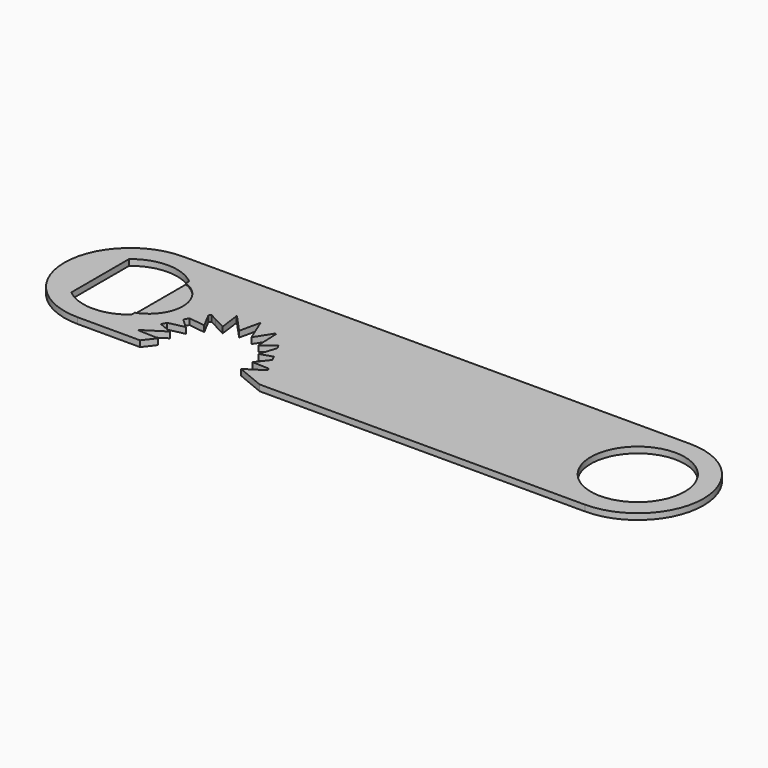
from build123d import *

# Parameters (mm, degrees)
F0_R     = 15.875
F1_DEPTH = 1.016
F3_DEPTH = 0.381


# Not quite as in the source:
# - a pattern or mirror of a feature is missing from the dataset's text; its kind, count and spacing are read off the source's solid
# - a feature names something its author has since deleted; it is built from what else it names


with BuildPart() as f1:
    # F0 (on Top) → F1 (new body, symmetric)
    with BuildSketch(Plane.XY):
        with BuildLine():
            Line((76.2, 22.225), (-95.25, 22.225))
            ThreePointArc((-95.25, 22.225), (-117.475, 0), (-95.25, -22.225))
            Line((-95.25, -22.225), (-81.2163393225, -22.225))
            Line((-81.2163393225, -22.225), (-80.4999828905, -20.8488920975))
            Line((-80.4999828905, -20.8488920975), (-81.8859980281, -17.8765730428))
            Line((-81.8859980281, -17.8765730428), (-80.3221061469, -17.944854037))
            Line((-80.3221061469, -17.944854037), (-81.0788131138, -9.2956538274))
            Line((-81.0788131138, -9.2956538274), (-79.6325889287, -9.8946994991))
            Line((-79.6325889287, -9.8946994991), (-77.3854601863, -1.5083008612))
            Line((-77.3854601863, -1.5083008612), (-76.231339678, -2.5658574615))
            Line((-76.231339678, -2.5658574615), (-71.2514121167, 4.5462161589))
            Line((-71.2514121167, 4.5462161589), (-70.5285992516, 3.1577055639))
            Line((-70.5285992516, 3.1577055639), (-63.4165256312, 8.1376331253))
            Line((-63.4165256312, 8.1376331253), (-63.2122023083, 6.5856434055))
            Line((-63.2122023083, 6.5856434055), (-54.8258036704, 8.832772148))
            Line((-54.8258036704, 8.832772148), (-55.1646142981, 7.3044961686))
            Line((-55.1646142981, 7.3044961686), (-46.5154140885, 6.5477892017))
            Line((-46.5154140885, 6.5477892017), (-47.3564931047, 5.2275596009))
            Line((-47.3564931047, 5.2275596009), (-39.4877125173, 1.5582869527))
            Line((-39.4877125173, 1.5582869527), (-40.7296133796, 0.6053429047))
            Line((-40.7296133796, 0.6053429047), (-34.5903434842, -5.5339269908))
            Line((-34.5903434842, -5.5339269908), (-36.0832746201, -6.0046463698))
            Line((-36.0832746201, -6.0046463698), (-32.4140019719, -13.8734269572))
            Line((-32.4140019719, -13.8734269572), (-33.9778938531, -13.805145963))
            Line((-33.9778938531, -13.805145963), (-33.273088024, -21.8611134529))
            Line((-33.273088024, -21.8611134529), (-33.0836606775, -22.225))
            Line((-33.0836606775, -22.225), (76.2, -22.225))
            ThreePointArc((76.2, -22.225), (98.425, 0), (76.2, 22.225))
        make_face()
        with BuildLine():
            ThreePointArc((-105.41, 12.1979516723), (-95.25, 15.875), (-85.09, 12.1979516723))
            Line((-85.09, 12.1979516723), (-85.09, -12.1979516723))
            ThreePointArc((-85.09, -12.1979516723), (-95.25, -15.875), (-105.41, -12.1979516723))
            Line((-105.41, -12.1979516723), (-105.41, 12.1979516723))
        make_face(mode=Mode.SUBTRACT)
        with Locations((76.2, 0)):
            Circle(F0_R, mode=Mode.SUBTRACT)
        Polygon((-80.4999828905, -20.8488920975), (-81.2163393225, -22.225), (-79.8582932371, -22.225), align=None)
        Polygon((-33.2412520763, -22.225), (-33.0836606775, -22.225), (-33.273088024, -21.8611134529), align=None)
        Polygon((-80.4999828905, -20.8488920975), (-79.8582932371, -22.225), (-77.6369016412, -22.225), (-74.1351559236, -22.225), (-71.1579054788, -18.3449716791), (-78.4147248097, -18.0281321046), (-79.3376725148, -18.6161146398), align=None)
        Polygon((-81.8859980281, -17.8765730428), (-80.4999828905, -20.8488920975), (-79.3376725148, -18.6161146398), (-80.2145068425, -19.1747197137), (-80.3221061469, -17.944854037), align=None)
        Polygon((-33.7748775265, -22.225), (-33.2412520763, -22.225), (-33.273088024, -21.8611134529), (-37.1054537581, -14.4992073738), (-43.1420945212, -18.3449716791), align=None)
        Polygon((-37.1054537581, -14.4992073738), (-33.273088024, -21.8611134529), (-33.9778938531, -13.805145963), (-35.8852751903, -13.7218678954), align=None)
        Polygon((-79.0178794125, -18.001797806), (-79.3376725148, -18.6161146398), (-78.4147248097, -18.0281321046), align=None)
        Polygon((-80.2145068425, -19.1747197137), (-79.3376725148, -18.6161146398), (-79.0178794125, -18.001797806), (-80.3221061469, -17.944854037), align=None)
        Polygon((-35.8852751903, -13.7218678954), (-33.9778938531, -13.805145963), (-34.0854931575, -12.5752802863), align=None)
        Polygon((-34.0854931575, -12.5752802863), (-33.9778938531, -13.805145963), (-32.4140019719, -13.8734269572), (-36.0832746201, -6.0046463698), (-37.9041095643, -6.5787534225), (-39.8848289883, -9.1600772324), (-37.5478999587, -13.6492761303), (-35.8852751903, -13.7218678954), align=None)
        Polygon((-37.5478999587, -13.6492761303), (-37.1054537581, -14.4992073738), (-35.8852751903, -13.7218678954), align=None)
        Polygon((-81.0788131138, -9.2956538274), (-80.3221061469, -17.944854037), (-79.0178794125, -18.001797806), (-75.6552159218, -11.5421813412), (-77.8687195378, -10.6253181231), (-79.9521174914, -11.0871963296), (-79.6325889287, -9.8946994991), align=None)
        Polygon((-79.0178794125, -18.001797806), (-78.4147248097, -18.0281321046), (-71.1579054788, -13.4050283209), (-75.6552159218, -11.5421813412), align=None)
        Polygon((-43.1420945212, -13.4050283209), (-37.5478999587, -13.6492761303), (-39.8848289883, -9.1600772324), align=None)
        Polygon((-77.8687195378, -10.6253181231), (-75.6552159218, -11.5421813412), (-74.8268774652, -9.950957971), align=None)
        Polygon((-37.9041095643, -6.5787534225), (-36.0832746201, -6.0046463698), (-36.6050237274, -4.8857517984), align=None)
        Polygon((-36.6050237274, -4.8857517984), (-36.0832746201, -6.0046463698), (-34.5903434842, -5.5339269908), (-40.7296133796, 0.6053429047), (-42.2442823639, -0.5569034849), (-43.0436234519, -3.0920895249), (-40.7598556276, -7.4791666976), (-37.9041095643, -6.5787534225), align=None)
        Polygon((-40.7598556276, -7.4791666976), (-39.8848289883, -9.1600772324), (-37.9041095643, -6.5787534225), align=None)
        Polygon((-77.8687195378, -10.6253181231), (-79.6325889287, -9.8946994991), (-79.9521174914, -11.0871963296), align=None)
        Polygon((-77.3854601863, -1.5083008612), (-79.6325889287, -9.8946994991), (-77.8687195378, -10.6253181231), (-74.8268774652, -9.950957971), (-72.6776090009, -5.822251665), (-74.8237309138, -3.855693253), (-76.9394562474, -3.5771527286), (-76.231339678, -2.5658574615), align=None)
        Polygon((-72.6776090009, -5.822251665), (-74.8268774652, -9.950957971), (-69.4683453434, -8.763), align=None)
        Polygon((-44.8316546566, -8.763), (-40.7598556276, -7.4791666976), (-43.0436234519, -3.0920895249), align=None)
        Polygon((-74.8237309138, -3.855693253), (-72.6776090009, -5.822251665), (-71.8571921171, -4.2462454947), align=None)
        Polygon((-42.2442823639, -0.5569034849), (-40.7296133796, 0.6053429047), (-41.6025816474, 1.4783111724), align=None)
        with BuildLine():
            Line((-41.6025816474, 1.4783111724), (-40.7296133796, 0.6053429047))
            Line((-40.7296133796, 0.6053429047), (-39.4877125173, 1.5582869527))
            Line((-39.4877125173, 1.5582869527), (-47.3564931047, 5.2275596009))
            Line((-47.3564931047, 5.2275596009), (-48.3823046954, 3.617357942))
            Line((-48.3823046954, 3.617357942), (-48.348249672, 2.8373696699))
            ThreePointArc((-48.348249672, 2.8373696699), (-45.8449546627, 0.7708533195), (-43.8143326805, -1.7616454653))
            Line((-43.8143326805, -1.7616454653), (-42.2442823639, -0.5569034849))
            Line((-42.2442823639, -0.5569034849), (-41.6025816474, 1.4783111724))
        make_face()
        with BuildLine():
            Line((-43.0687030233, -3.0439121166), (-43.0436234519, -3.0920895249))
            Line((-43.0436234519, -3.0920895249), (-42.2442823639, -0.5569034849))
            Line((-42.2442823639, -0.5569034849), (-43.8143326805, -1.7616454653))
            ThreePointArc((-43.8143326805, -1.7616454653), (-43.4265334283, -2.3940654467), (-43.0687030233, -3.0439121166))
        make_face()
        Polygon((-74.8237309138, -3.855693253), (-76.231339678, -2.5658574615), (-76.9394562474, -3.5771527286), align=None)
        with BuildLine():
            Line((-71.2514121167, 4.5462161589), (-76.231339678, -2.5658574615))
            Line((-76.231339678, -2.5658574615), (-74.8237309138, -3.855693253))
            Line((-74.8237309138, -3.855693253), (-71.8571921171, -4.2462454947))
            Line((-71.8571921171, -4.2462454947), (-71.2312969767, -3.0439121166))
            ThreePointArc((-71.2312969767, -3.0439121166), (-70.2116133855, -1.3514289323), (-68.9895778341, 0.2012729279))
            Line((-68.9895778341, 0.2012729279), (-69.6470295052, 1.4642258374))
            Line((-69.6470295052, 1.4642258374), (-71.5398945187, 2.4495889946))
            Line((-71.5398945187, 2.4495889946), (-70.5285992516, 3.1577055639))
            Line((-70.5285992516, 3.1577055639), (-71.2514121167, 4.5462161589))
        make_face()
        with BuildLine():
            Line((-71.2312969767, -3.0439121166), (-71.8571921171, -4.2462454947))
            Line((-71.8571921171, -4.2462454947), (-66.2930109602, -4.9787838411))
            Line((-66.2930109602, -4.9787838411), (-68.9895778341, 0.2012729279))
            ThreePointArc((-68.9895778341, 0.2012729279), (-70.2116133855, -1.3514289323), (-71.2312969767, -3.0439121166))
        make_face()
        Polygon((-48.3823046954, 3.617357942), (-47.3564931047, 5.2275596009), (-48.4753876761, 5.7493087082), align=None)
        with BuildLine():
            Line((-48.4753876761, 5.7493087082), (-47.3564931047, 5.2275596009))
            Line((-47.3564931047, 5.2275596009), (-46.5154140885, 6.5477892017))
            Line((-46.5154140885, 6.5477892017), (-55.1646142981, 7.3044961686))
            Line((-55.1646142981, 7.3044961686), (-55.5778404781, 5.4405533245))
            Line((-55.5778404781, 5.4405533245), (-55.5701648333, 5.4220226787))
            ThreePointArc((-55.5701648333, 5.4220226787), (-52.0121003071, 4.6464015983), (-48.7243991788, 3.0803771655))
            Line((-48.7243991788, 3.0803771655), (-48.3823046954, 3.617357942))
            Line((-48.3823046954, 3.617357942), (-48.4753876761, 5.7493087082))
        make_face()
        with BuildLine():
            Line((-48.0069890398, -4.9787838411), (-43.8143326805, -1.7616454653))
            ThreePointArc((-43.8143326805, -1.7616454653), (-45.8449546627, 0.7708533195), (-48.348249672, 2.8373696699))
            Line((-48.348249672, 2.8373696699), (-48.2236044906, -0.017474342))
            Line((-48.2236044906, -0.017474342), (-48.0069890398, -4.9787838411))
        make_face()
        Polygon((-69.6470295052, 1.4642258374), (-70.5285992516, 3.1577055639), (-71.5398945187, 2.4495889946), align=None)
        with BuildLine():
            Line((-63.4165256312, 8.1376331253), (-70.5285992516, 3.1577055639))
            Line((-70.5285992516, 3.1577055639), (-69.6470295052, 1.4642258374))
            Line((-69.6470295052, 1.4642258374), (-68.4074402589, 0.8189365196))
            ThreePointArc((-68.4074402589, 0.8189365196), (-65.8542771411, 2.9017913046), (-62.9261305575, 4.4127127279))
            Line((-62.9261305575, 4.4127127279), (-62.9630019017, 4.6927783921))
            Line((-62.9630019017, 4.6927783921), (-64.4046991388, 6.2661148428))
            Line((-64.4046991388, 6.2661148428), (-63.2122023083, 6.5856434055))
            Line((-63.2122023083, 6.5856434055), (-63.4165256312, 8.1376331253))
        make_face()
        with BuildLine():
            Line((-69.6470295052, 1.4642258374), (-68.9895778341, 0.2012729279))
            ThreePointArc((-68.9895778341, 0.2012729279), (-68.7026377194, 0.5139959287), (-68.4074402589, 0.8189365196))
            Line((-68.4074402589, 0.8189365196), (-69.6470295052, 1.4642258374))
        make_face()
        with BuildLine():
            Line((-48.348249672, 2.8373696699), (-48.3823046954, 3.617357942))
            Line((-48.3823046954, 3.617357942), (-48.7243991788, 3.0803771655))
            ThreePointArc((-48.7243991788, 3.0803771655), (-48.5354675075, 2.9601998346), (-48.348249672, 2.8373696699))
        make_face()
        with BuildLine():
            ThreePointArc((-62.9261305575, 4.4127127279), (-65.8542771411, 2.9017913046), (-68.4074402589, 0.8189365196))
            Line((-68.4074402589, 0.8189365196), (-66.2308278804, -0.3141361665))
            Line((-66.2308278804, -0.3141361665), (-62.0148945187, -2.5088121619))
            Line((-62.0148945187, -2.5088121619), (-62.9261305575, 4.4127127279))
        make_face()
        with BuildLine():
            Line((-56.3944799748, 7.412095473), (-55.1646142981, 7.3044961686))
            Line((-55.1646142981, 7.3044961686), (-54.8258036704, 8.832772148))
            Line((-54.8258036704, 8.832772148), (-63.2122023083, 6.5856434055))
            Line((-63.2122023083, 6.5856434055), (-62.9630019017, 4.6927783921))
            Line((-62.9630019017, 4.6927783921), (-62.7636045656, 4.4751743841))
            ThreePointArc((-62.7636045656, 4.4751743841), (-59.2274466598, 5.3643114334), (-55.5816939364, 5.4231714974))
            Line((-55.5816939364, 5.4231714974), (-55.5778404781, 5.4405533245))
            Line((-55.5778404781, 5.4405533245), (-56.3944799748, 7.412095473))
        make_face()
        Polygon((-55.5778404781, 5.4405533245), (-55.1646142981, 7.3044961686), (-56.3944799748, 7.412095473), align=None)
        with BuildLine():
            Line((-52.2851054813, -2.5088121619), (-48.7243991788, 3.0803771655))
            ThreePointArc((-48.7243991788, 3.0803771655), (-52.0121003071, 4.6464015983), (-55.5701648333, 5.4220226787))
            Line((-55.5701648333, 5.4220226787), (-52.2851054813, -2.5088121619))
        make_face()
        Polygon((-62.9630019017, 4.6927783921), (-63.2122023083, 6.5856434055), (-64.4046991388, 6.2661148428), align=None)
        with BuildLine():
            Line((-62.9630019017, 4.6927783921), (-62.9261305575, 4.4127127279))
            ThreePointArc((-62.9261305575, 4.4127127279), (-62.8449531963, 4.4441663787), (-62.7636045656, 4.4751743841))
            Line((-62.7636045656, 4.4751743841), (-62.9630019017, 4.6927783921))
        make_face()
        with BuildLine():
            Line((-55.5701648333, 5.4220226787), (-55.5778404781, 5.4405533245))
            Line((-55.5778404781, 5.4405533245), (-55.5816939364, 5.4231714974))
            ThreePointArc((-55.5816939364, 5.4231714974), (-55.57592928, 5.4225981398), (-55.5701648333, 5.4220226787))
        make_face()
        with BuildLine():
            ThreePointArc((-55.5816939364, 5.4231714974), (-59.2274466598, 5.3643114334), (-62.7636045656, 4.4751743841))
            Line((-62.7636045656, 4.4751743841), (-57.15, -1.651))
            Line((-57.15, -1.651), (-55.5816939364, 5.4231714974))
        make_face()
    extrude(amount=F1_DEPTH, both=True)

    # F2 (on face) → F3 (cut)
    with BuildSketch(Plane.XY.offset(1.016)):
        with BuildLine():
            ThreePointArc((-85.09, -10.7763073453), (-79.56744408, -6.5991135768), (-77.47, 0))
            ThreePointArc((-77.47, 0), (-79.56744408, 6.5991135768), (-85.09, 10.7763073453))
            Line((-85.09, 10.7763073453), (-85.09, -10.7763073453))
        make_face()
    f3 = extrude(amount=-F3_DEPTH, mode=Mode.SUBTRACT)

    # F3_copies: F3 across plane
    add(f3.mirror(Plane(origin=(0, 0, 0), x_dir=(-1, 0, 0), z_dir=(0, 0, -1))), mode=Mode.SUBTRACT)


solid = f1.part
